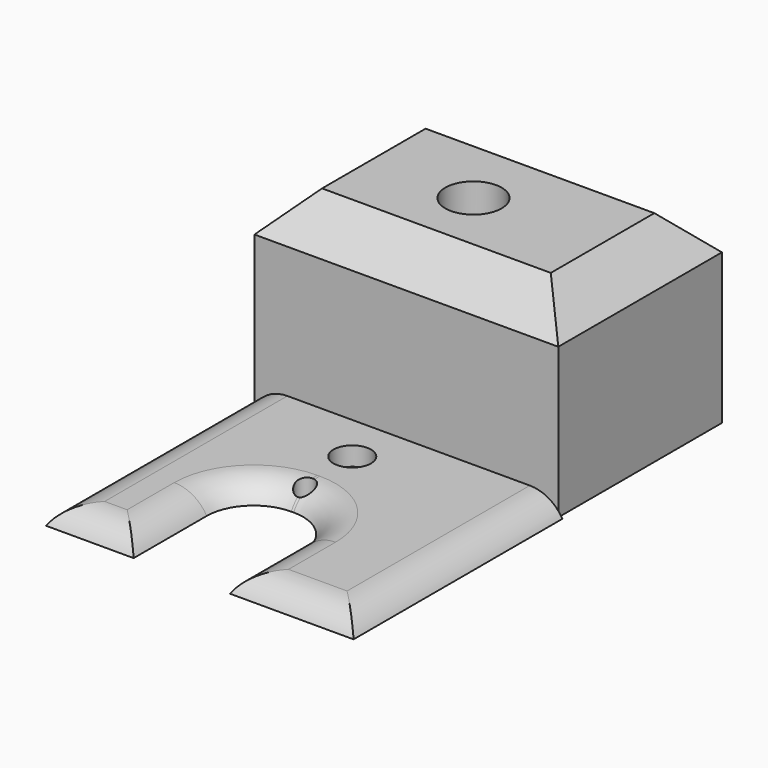
from build123d import *

# Parameters (mm, degrees)
F0_W          = 41.1070454866
F0_H          = 27.6698879898
F1_DEPTH      = 25.4
F2_W          = 41.600080207
F2_H          = 35.3044494987
F3_DEPTH      = 2.54
F5_DEPTH      = 25.4
F7_D          = 7.62
F7_DEPTH      = 508
F7_TIP        = 2.2892789585
F9_D          = 2.54
F9_DEPTH      = 508
F9_TIP        = 0.7630929862
F11_D         = 5.08
F11_DEPTH     = 508
F11_TIP       = 1.5261859723
F12_SIZE      = 5.08
F13_T1_DEPTH  = 46.3029721267
F13_T3_DEPTH  = 38.7218051595
F13_T5_DEPTH  = 33.8444602975
F13_T7_DEPTH  = 23.3607587036
F13_T9_DEPTH  = 0.3279052623
F13_T12_ANGLE = 90
F13_T14_ANGLE = 90


# Not quite as in the source:
# - a fillet or chamfer that OpenCascade refuses, or shapes differently, is made with other operations: its cross-section is extruded or revolved along the edge and cut away or added


with BuildPart() as f1:
    # F0 (on Top) → F1 (new body)
    with BuildSketch(Plane.XY):
        with Locations((-4.3705804273, 13.8349439949)):
            Rectangle(F0_W, F0_H)
    extrude(amount=F1_DEPTH)

    # F2 (on Top) → F3 (join)
    with BuildSketch(Plane.XY):
        with Locations((-4.0700184181, -17.6522247493)):
            Rectangle(F2_W, F2_H)
    extrude(amount=F3_DEPTH)

    # F4 (on face) → F5 (cut)
    with BuildSketch(Plane.XY.offset(2.54)):
        with BuildLine():
            Line((-13.0226434802, -22.9422134231), (-13.0226434802, -45.534973538))
            Line((-13.0226434802, -45.534973538), (0.005261782, -45.534973538))
            Line((0.005261782, -45.534973538), (0.005261782, -22.9422134231))
            ThreePointArc((0.005261782, -22.9422134231), (-1.8546101574, -18.4520853626), (-6.344738218, -16.5922134231))
            Line((-6.344738218, -16.5922134231), (-6.6726434802, -16.5922134231))
            ThreePointArc((-6.6726434802, -16.5922134231), (-11.1627715408, -18.4520853626), (-13.0226434802, -22.9422134231))
        make_face()
    extrude(amount=-F5_DEPTH, mode=Mode.SUBTRACT)

    # F7
    with Locations(Plane.XY.offset(25.4)):
        with Locations((-5.9787402861, 13.3550977334)):
            Hole(F7_D / 2, depth=F7_DEPTH)
            with Locations((0, 0, -(F7_DEPTH + F7_TIP / 2))):  # 118° drill point
                Cone(0, F7_D / 2, F7_TIP, mode=Mode.SUBTRACT)

    # F9
    with Locations(Plane.XY.offset(2.54)):
        with Locations((-6.6726434802, -14.2427943647)):
            Hole(F9_D / 2, depth=F9_DEPTH)
            with Locations((0, 0, -(F9_DEPTH + F9_TIP / 2))):  # 118° drill point
                Cone(0, F9_D / 2, F9_TIP, mode=Mode.SUBTRACT)

    # F11
    with Locations(Plane.XY.offset(2.54)):
        with Locations((-6.4694355242, -6.5277060494)):
            Hole(F11_D / 2, depth=F11_DEPTH)
            with Locations((0, 0, -(F11_DEPTH + F11_TIP / 2))):  # 118° drill point
                Cone(0, F11_D / 2, F11_TIP, mode=Mode.SUBTRACT)

    # F12
    f12_edges = [f1.edges().sort_by_distance(p)[0] for p in [
        (-4.37058, 0, 25.4),
        (16.182942, 13.834944, 25.4),
        (-4.37058, 27.669888, 25.4),
        (-24.924103, 13.834944, 25.4),
    ]]
    chamfer(f12_edges, length=F12_SIZE)

    # F13: fillet of radius 5.08 on 5 edges, made by hand

    # F13_s2 → F13_t1 (cut)
    with BuildSketch(Plane.XZ):
        with BuildLine():
            ThreePointArc((16.7300216854, 0), (14.8706126341, 1.8594090512), (12.3306126341, 2.54))
            Line((12.3306126341, 2.54), (16.7300216854, 2.54))
            Line((16.7300216854, 2.54), (16.7300216854, 0))
        make_face()
        with BuildLine():
            ThreePointArc((-24.8700585216, 0), (-23.0106494704, 1.8594090512), (-20.4706494704, 2.54))
            Line((-20.4706494704, 2.54), (-24.8700585216, 2.54))
            Line((-24.8700585216, 2.54), (-24.8700585216, 0))
        make_face()
    extrude(amount=F13_T1_DEPTH, mode=Mode.SUBTRACT)

    # F13_s4 → F13_t3 (cut)
    with BuildSketch(Plane.YZ.offset(-10.993260846)):
        with BuildLine():
            ThreePointArc((-35.3044494987, 0), (-33.4450404474, 1.8594090512), (-30.9050404474, 2.54))
            Line((-30.9050404474, 2.54), (-35.3044494987, 2.54))
            Line((-35.3044494987, 2.54), (-35.3044494987, 0))
        make_face()
    extrude(amount=F13_T3_DEPTH, mode=Mode.SUBTRACT)

    # F13_s6 → F13_t5 (cut)
    with BuildSketch(Plane.YZ.offset(-35.8685811497)):
        with BuildLine():
            ThreePointArc((-35.3044494987, 0), (-33.4450404474, 1.8594090512), (-30.9050404474, 2.54))
            Line((-30.9050404474, 2.54), (-35.3044494987, 2.54))
            Line((-35.3044494987, 2.54), (-35.3044494987, 0))
        make_face()
    extrude(amount=F13_T5_DEPTH, mode=Mode.SUBTRACT)

    # F13_s8 → F13_t7 (cut)
    with BuildSketch(Plane.XZ.offset(22.9422134231)):
        with BuildLine():
            ThreePointArc((0.005261782, 0), (1.8646708333, 1.8594090512), (4.4046708333, 2.54))
            Line((4.4046708333, 2.54), (0.005261782, 2.54))
            Line((0.005261782, 2.54), (0.005261782, 0))
        make_face()
        with BuildLine():
            ThreePointArc((-13.0226434802, 0), (-14.8820525315, 1.8594090512), (-17.4220525315, 2.54))
            Line((-17.4220525315, 2.54), (-13.0226434802, 2.54))
            Line((-13.0226434802, 2.54), (-13.0226434802, 0))
        make_face()
    extrude(amount=F13_T7_DEPTH, mode=Mode.SUBTRACT)

    # F13_s10 → F13_t9 (cut)
    with BuildSketch(Plane.YZ.offset(-6.6726434802)):
        with BuildLine():
            ThreePointArc((-16.5922134231, 0), (-14.7328043719, 1.8594090512), (-12.1928043719, 2.54))
            Line((-12.1928043719, 2.54), (-16.5922134231, 2.54))
            Line((-16.5922134231, 2.54), (-16.5922134231, 0))
        make_face()
    extrude(amount=F13_T9_DEPTH, mode=Mode.SUBTRACT)

    # F13_s11 → F13_t12 (revolve, cut)
    with BuildSketch(Plane.XZ.offset(22.9422134231)):
        with BuildLine():
            ThreePointArc((0.005261782, 0), (1.8646708333, 1.8594090512), (4.4046708333, 2.54))
            Line((4.4046708333, 2.54), (0.005261782, 2.54))
            Line((0.005261782, 2.54), (0.005261782, 0))
        make_face()
    revolve(axis=Axis((-6.344738218, -22.9422134231, 2.54), (0, 0, 1)), revolution_arc=F13_T12_ANGLE, mode=Mode.SUBTRACT)

    # F13_s13 → F13_t14 (revolve, cut)
    with BuildSketch(Plane.YZ.offset(-6.6726434802)):
        with BuildLine():
            ThreePointArc((-16.5922134231, 0), (-14.7328043719, 1.8594090512), (-12.1928043719, 2.54))
            Line((-12.1928043719, 2.54), (-16.5922134231, 2.54))
            Line((-16.5922134231, 2.54), (-16.5922134231, 0))
        make_face()
    revolve(axis=Axis((-6.6726434802, -22.9422134231, 2.54), (0, 0, 1)), revolution_arc=F13_T14_ANGLE, mode=Mode.SUBTRACT)


solid = f1.part
